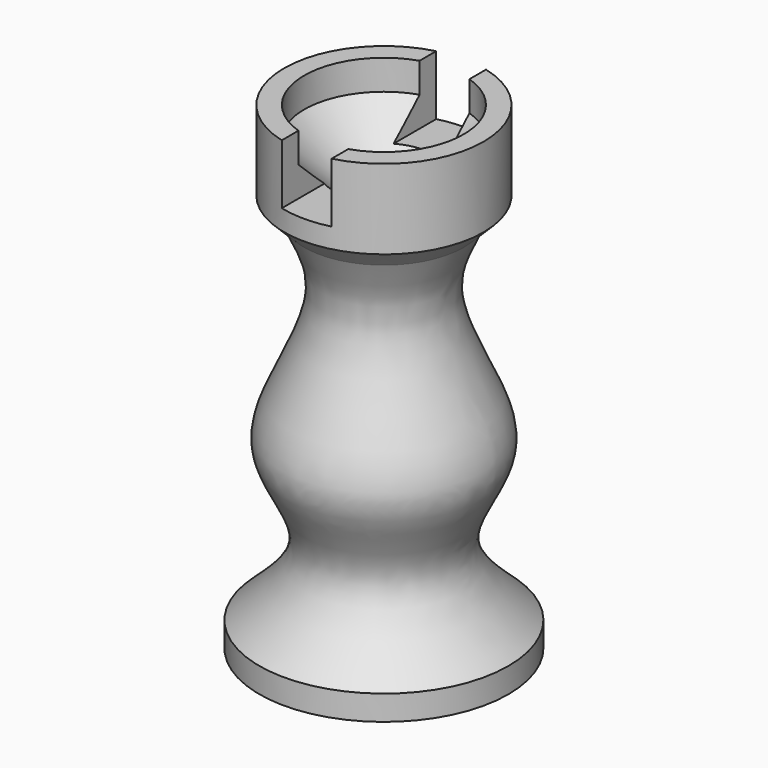
from build123d import *

# Parameters (mm, degrees)
F0_W     = 12.5
F0_H     = 2.5
F2_W     = 5
F2_H     = 30
F3_DEPTH = 6


# Not quite as in the source:
# - a fillet or chamfer that OpenCascade refuses, or shapes differently, is made with other operations: its cross-section is extruded or revolved along the edge and cut away or added


with BuildPart() as f1:
    # F0 (on Front) → F1 (revolve)
    with BuildSketch(Plane.XZ):
        with BuildLine():
            Line((0, 2.5), (12.5, 2.5))
            add(Edge.make_bspline(
                [(8, 38), (7.0575290046, 36.0296102259), (4.9176459622, 31.9169764445), (8.8571855748, 23.8819266131), (11.7311727266, 17.2522437772), (5.0634432181, 9.5532988579), (9.6973287885, 5.0417102196), (12.5, 2.5)],
                knots=[0, 0, 0, 0, 0.1821407595, 0.3923850866, 0.5803644457, 0.7831417696, 1, 1, 1, 1], degree=3))
            Line((8, 38), (0, 38))
            Line((0, 38), (0, 2.5))
        make_face()
        with Locations((6.25, 1.25)):
            Rectangle(F0_W, F0_H)
        Polygon((10, 40), (10, 48), (8, 48), (8, 40), (0, 40), (0, 38), (8, 38), align=None)
    revolve(axis=Axis((0, 0, 44), (0, 0, -1)))

    # F2 (on face) → F3 (cut)
    with BuildSketch(Plane.XY.offset(48)):
        Rectangle(F2_W, F2_H)
    extrude(amount=-F3_DEPTH, mode=Mode.SUBTRACT)

    # F4: chamfer of 5 on 1 edges, made by hand


with BuildPart() as f4_tool2:
    # F4_s3 → F4_t4 (revolve)
    with BuildSketch(Plane.XZ):
        Polygon((8, 45), (3, 40), (8, 40), align=None)
    revolve(axis=Axis((0, 0, 40), (0, 0, -1)))

    split(bisect_by=Plane.YZ.offset(2.5), keep=Keep.TOP)


with BuildPart() as f1_1:
    add(f1.part)

    # F4_t1: union F4_tool2
    add(f4_tool2.part)


with BuildPart() as f4_tool7:
    # F4_s8 → F4_t9 (revolve)
    with BuildSketch(Plane.XZ):
        Polygon((8, 45), (3, 40), (8, 40), align=None)
    revolve(axis=Axis((0, 0, 40), (0, 0, -1)))

    split(bisect_by=Plane.XY.offset(42), keep=Keep.BOTTOM)


with BuildPart() as f1_2:
    add(f1_1.part)

    # F4_t6: union F4_tool7
    add(f4_tool7.part)


with BuildPart() as f4_tool12:
    # F4_s13 → F4_t14 (revolve)
    with BuildSketch(Plane.XZ):
        Polygon((8, 45), (3, 40), (8, 40), align=None)
    revolve(axis=Axis((0, 0, 40), (0, 0, -1)))

    split(bisect_by=Plane.YZ.offset(-2.5), keep=Keep.BOTTOM)


with BuildPart() as f1_3:
    add(f1_2.part)

    # F4_t11: union F4_tool12
    add(f4_tool12.part)


solid = f1_3.part
